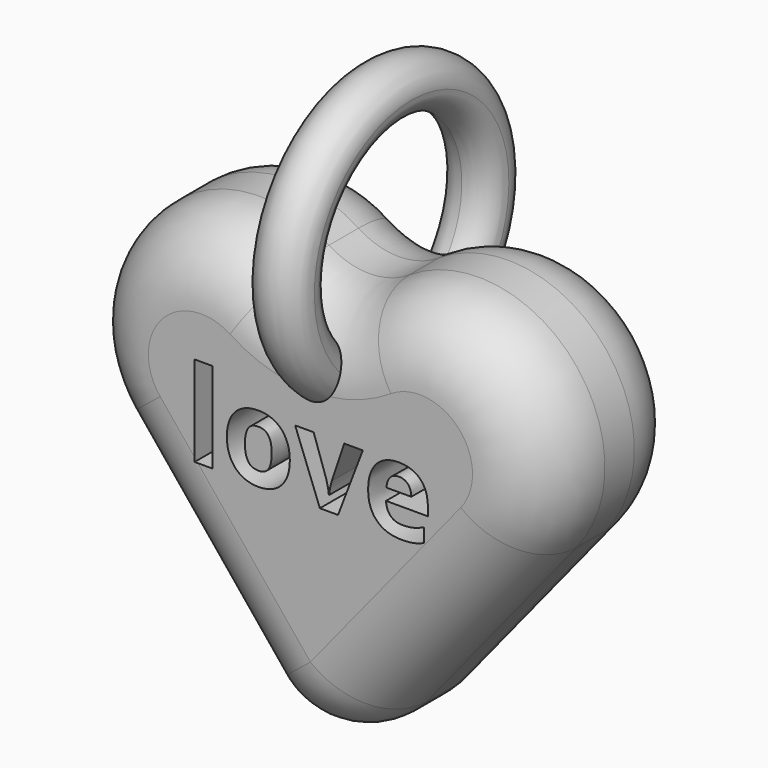
from build123d import *

# Parameters (mm, degrees)
F1_DEPTH     = 12.7
F2_R         = 5.08
F3_TEXT_SIZE = 8.2080976831
F4_DEPTH     = 3.81


# Not quite as in the source:
# - Text() gives the source's letters only with a copy of the font that has no kerning and outlines rounded to 1/6400 em; it was checked with that copy


with BuildPart() as f1:
    # F0 (on Front) → F1 (new body)
    with BuildSketch(Plane.XZ):
        with BuildLine():
            Line((-14.3199730664, 0), (0, -17.6158379763))
            Line((0, -17.6158379763), (14.3199730664, 0))
            ThreePointArc((14.3199730664, 0), (12.5066257593, 12.687209061), (0, 9.8875993863))
            ThreePointArc((0, 9.8875993863), (-12.5066257593, 12.687209061), (-14.3199730664, 0))
        make_face()
    extrude(amount=F1_DEPTH)

    # F2
    f2_edges = [f1.edges().sort_by_distance(p)[0] for p in [
        (0, -6.35, -17.615838),
        (14.319973, -6.35, 0),
        (7.159987, 0, -8.807919),
        (7.159987, -12.7, -8.807919),
        (0, -6.35, 9.887599),
        (12.506626, 0, 12.687209),
        (12.506626, -12.7, 12.687209),
        (-12.506626, 0, 12.687209),
        (-12.506626, -12.7, 12.687209),
    ]]
    fillet(f2_edges, radius=F2_R)

    # F3 (on face) → F4 (cut)
    with BuildSketch(Plane.XZ.offset(12.7)):
        with Locations((-8.6428703572, 0)):
            Text('love', F3_TEXT_SIZE, font='Open Sans', font_style=FontStyle.BOLD, text_align=(TextAlign.LEFT, TextAlign.BOTTOM))
    extrude(amount=-F4_DEPTH, mode=Mode.SUBTRACT)

    # F8: sweep along a path in F5
    with BuildLine(Plane.YZ) as f8_path:
        CenterArc((-6.3499999233, 14.245021157), 7.62, 0, 360)
    # F7 (on offset) → F8 (sweep)
    with BuildSketch(Plane.XY.offset(17.78)):
        with BuildLine():
            ThreePointArc((0, -12.0649999233), (-1.3470384182, -15.3170383414), (1.905, -13.9699999233))
            ThreePointArc((1.905, -13.9699999233), (1.3470384182, -12.6229615051), (0, -12.0649999233))
        make_face()
    sweep(path=f8_path.line)


solid = f1.part
